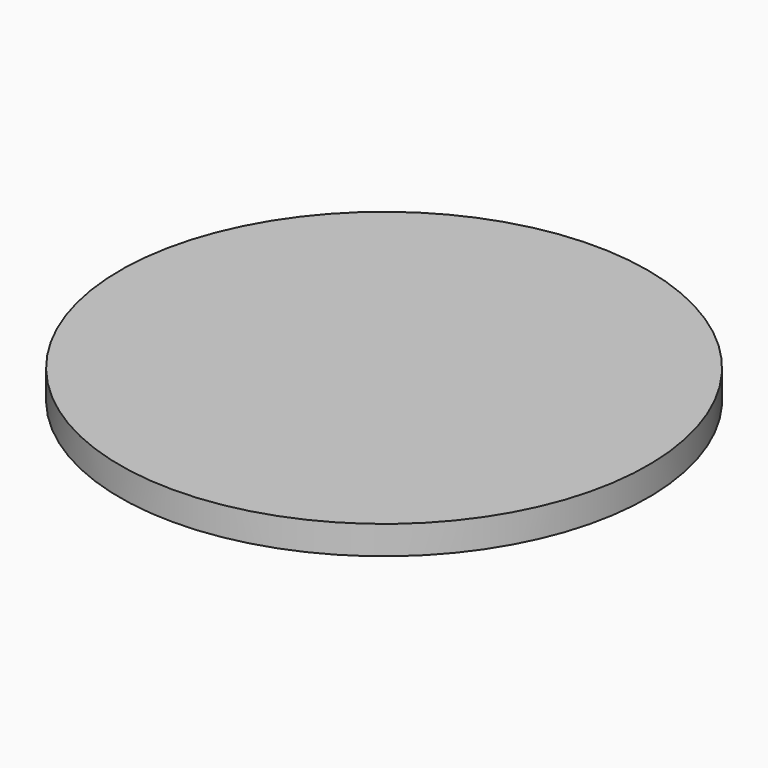
from build123d import *


# Not quite as in the source:
# - the dataset's text gives a spline's control points without its knots; the knots are read off the source's solid


with BuildPart() as f1:
    # F0 (on Right) → F1 (revolve)
    with BuildSketch(Plane.YZ):
        with BuildLine():
            Line((0, 20.6559349321), (-176, 20.6559349321))
            Line((-176, 20.6559349321), (-176, 1.6559349321))
            Line((-176, 1.6559349321), (-97, 1.6559349321))
            Line((-97, 1.6559349321), (-97, 8.6650897047))
            Line((-97, 8.6650897047), (-92, 8.6650897047))
            Line((-92, 8.6650897047), (-80.8910141144, 8.5638507627))
            ThreePointArc((-80.8910141144, 8.5638507627), (-78.9814421484, 14.1909154974), (-73.166703328, 15.4153072123))
            add(Edge.make_bspline(
                [(-73.1667033281, 15.4153072121), (-72.9471329023, 15.3448479619), (-72.4144283404, 15.1855308243), (-71.6023892617, 14.9948791803), (-70.4927976129, 14.7957954824), (-68.9835687024, 14.5469124184), (-67.0900004145, 14.2515001799), (-64.8292404487, 13.9210636753), (-62.2173324139, 13.5648597249), (-59.2706251911, 13.1927189393), (-56.0050605257, 12.8143593072), (-52.4377790806, 12.4393414695), (-48.581476538, 12.0779460108), (-43.1019911307, 11.6217131069), (-35.744340035, 11.1089813664), (-26.4785158191, 10.6187123314), (-17.1545160942, 10.2858528365), (-8.1509876938, 10.1427621339), (-2.6151021529, 10.1952662098), (-0.0277993408, 10.2637089327)],
                knots=[0.3243164972, 0.3243164972, 0.3243164972, 0.3243164972, 0.34375, 0.375, 0.40625, 0.4375, 0.46875, 0.5, 0.53125, 0.5625, 0.59375, 0.625, 0.65625, 0.6875, 0.75, 0.8125, 0.875, 0.9375, 0.99999, 0.99999, 0.99999, 0.99999], degree=3))
            Line((-0.0277993408, 10.2637089327), (0, 10.2637089327))
            Line((0, 10.2637089327), (0, 20.6559349321))
        make_face()
    revolve(axis=Axis((0, 0, 16.6838523), (0, 0, -1)))


solid = f1.part
